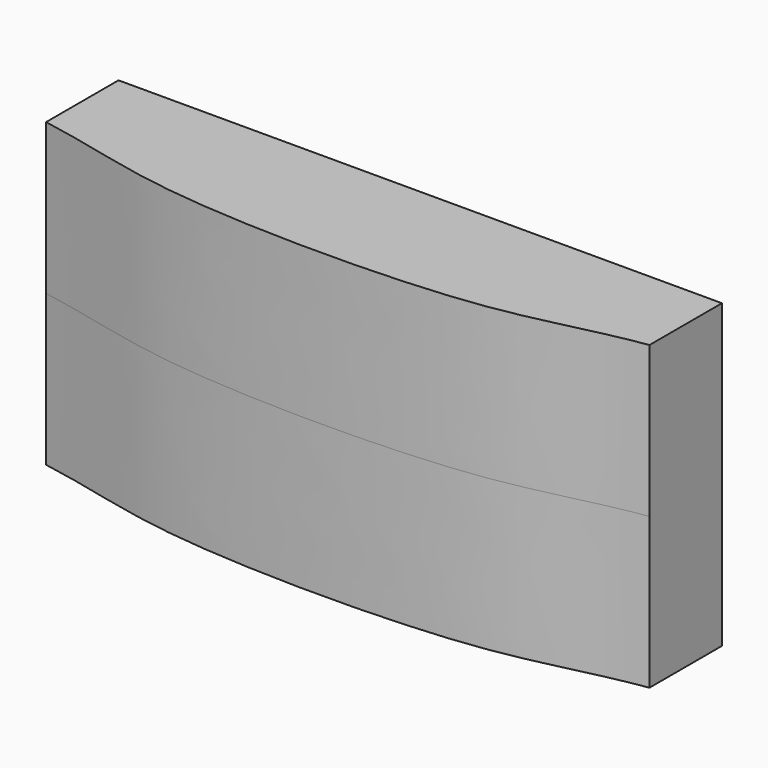
from build123d import *

# Parameters (mm, degrees)
F1_DEPTH = 25
F2_T     = -2.5
F3_R     = 6.6355388612
F3_R_2   = 4.1355388612
F4_DEPTH = 10


with BuildPart() as f1:
    # F0 (on Top) → F1 (new body, symmetric)
    with BuildSketch(Plane.XY):
        with BuildLine():
            Line((50, 10), (-50, 10))
            Line((-50, 10), (-50, -5))
            add(Edge.make_bspline(
                [(-50, -5), (-41.2109963008, -6.5224078765), (-26.5740678263, -11.7899728285), (26.9379984195, -11.8136836371), (40.5056804928, -6.4935245034), (50, -5)],
                knots=[0, 0, 0, 0, 0.2940817771, 0.7059182229, 1, 1, 1, 1], degree=3))
            Line((50, -5), (50, 10))
        make_face()
    extrude(amount=F1_DEPTH, both=True)

    # F2
    f2_openings = [f1.faces().sort_by_distance(p)[0] for p in [
        (0, 10, 0),
    ]]
    offset(amount=F2_T, openings=f2_openings, kind=Kind.INTERSECTION)



with BuildPart() as f4:
    # F3 (on Front) → F4 (new body, through all)
    with BuildSketch(Plane.XZ):
        with Locations((43.3644611388, -18.3644611388)):
            Circle(F3_R)
        with Locations((43.3644611388, -18.3644611388)):
            Circle(F3_R_2, mode=Mode.SUBTRACT)
    extrude(amount=-F4_DEPTH)


with BuildPart() as f5_1:
    # F5: instance of F4
    add(f4.part.mirror(Plane.XY))


with BuildPart() as f1_1:
    add(f1.part)

    add(f4.part)  # F6 merges F4

    add(f5_1.part)  # F6 merges F5_1
    # F6: F4, F5_1 across plane
    add(f4.part.mirror(Plane.YZ))
    add(f5_1.part.mirror(Plane.YZ))


solid = f1_1.part
